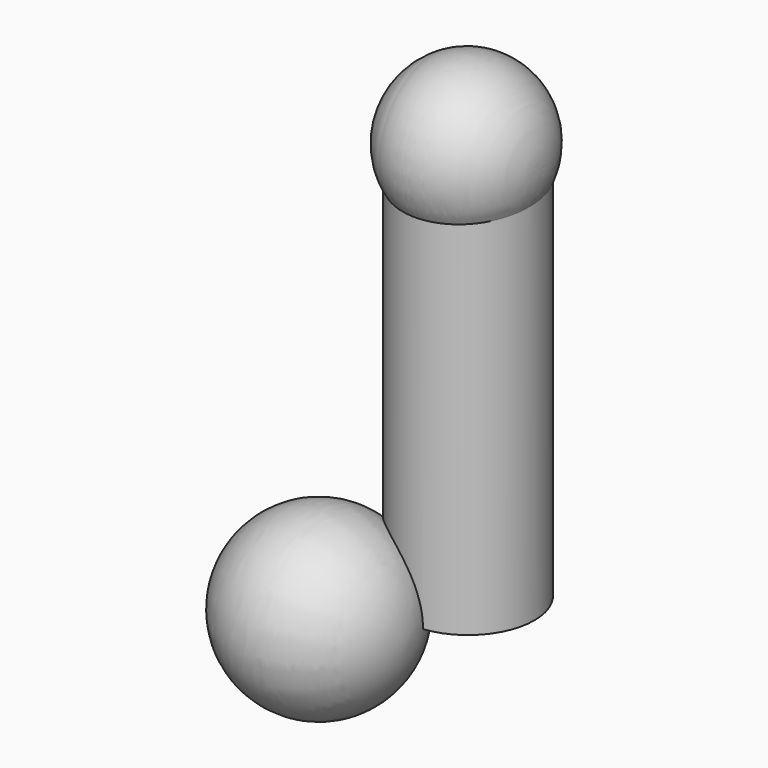
from build123d import *

# Parameters (mm, degrees)
F4_R     = 19.9281081923
F5_DEPTH = 120


# Not quite as in the source:
# - the program builds the solid bodies; features that only make, move or delete a surface that nothing else refers to are left out


with BuildPart() as f1:
    # F0 (on Top) → F1 (revolve)
    with BuildSketch(Plane.XY):
        with BuildLine():
            Line((-62.9295191233, 0.0105900164), (-10.0940960217, 0))
            ThreePointArc((-10.0940960217, 0), (-36.5065136255, 26.4177120814), (-62.9295191233, 0.0105900164))
        make_face()
    revolve(axis=Axis((-36.5118075725, 0.0052950082, 0), (0.9999999799, -0.000200434, 0)))

    # F4 (on Top) → F5 (join)
    with BuildSketch(Plane.XY):
        with Locations((-13.4765654802, 27.1572843194)):
            Circle(F4_R)
    extrude(amount=F5_DEPTH)

    # F6 (on face) → F7 (revolve)
    with BuildSketch(Plane.XY.offset(120)):
        with BuildLine():
            Line((-35.4603284685, 26.4999073577), (8.507197508, 26.4999073577))
            ThreePointArc((8.507197508, 26.4999073577), (-13.4765654802, 49.1508738307), (-35.4603284685, 26.4999073577))
        make_face()
    revolve(axis=Axis((-13.4765654802, 26.4999073577, 120), (1, 0, 0)))


solid = f1.part
